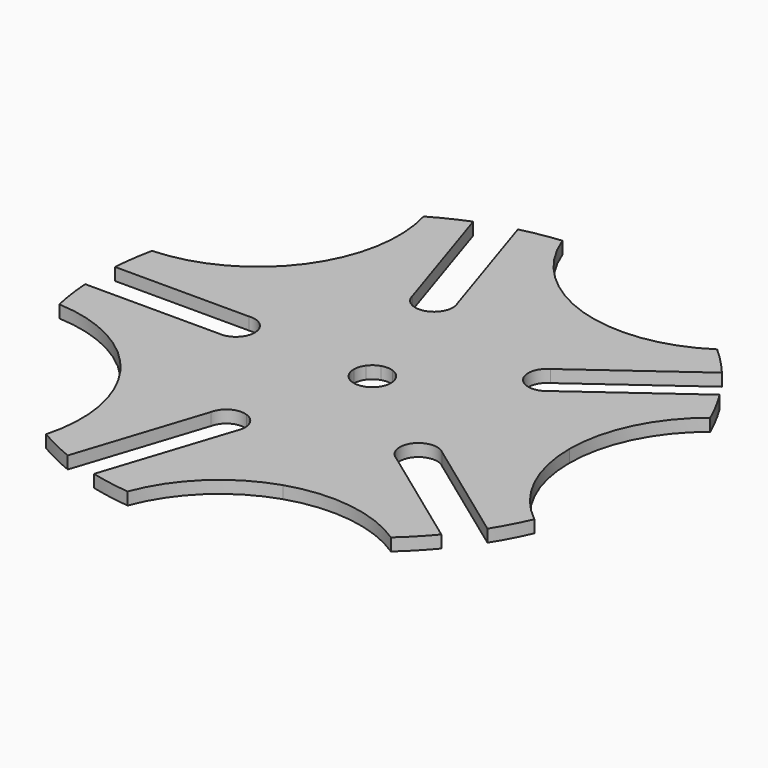
from build123d import *

# Parameters (mm, degrees)
F1_DEPTH = 3.175


# Not quite as in the source:
# - a length typed as a fraction of an inch, garbled in the dataset ("3 / 203.2 mm" for 3/8 in), is restored


with BuildPart() as f1:
    # F0 (on Top) → F1 (new body)
    with BuildSketch(Plane.XY):
        with BuildLine():
            ThreePointArc((-4.7624995714, 0.0020204955), (-4.528844398, 1.4734227733), (-3.8519931198, 2.800634795))
            Line((-3.8519931198, 2.800634795), (-40.7900391434, 29.6568553891))
            ThreePointArc((-40.7900391434, 29.6568553891), (-52.8581727457, 19.1196962374), (-68.3027796686, 14.8610945149))
            ThreePointArc((-68.3027796686, 14.8610945149), (-69.202037382, 9.8589990779), (-69.7354707037, 4.8047857774))
            Line((-69.7354707037, 4.8047857774), (-35.4708737874, 4.7902489857))
            ThreePointArc((-35.4708737874, 4.7902489857), (-31.7421994573, 3.5901618172), (-30.1466961845, 0.012789768))
            Line((-30.1466961845, 0.012789768), (-4.7624995714, 0.0020204955))
        make_face()
        with BuildLine():
            ThreePointArc((-3.8519931198, 2.800634795), (-2.7981829099, 3.853774598), (-1.4705404248, 4.5297811326))
            Line((-1.4705404248, 4.5297811326), (-9.3085437064, 28.6735848558))
            ThreePointArc((-9.3085437064, 28.6735848558), (-13.2035838045, 29.0881739368), (-15.4950023114, 32.2650627762))
            Line((-15.4950023114, 32.2650627762), (-26.0750504874, 64.8553280982))
            ThreePointArc((-26.0750504874, 64.8553280982), (-30.7184565015, 62.789316534), (-35.1994748016, 60.3913802983))
            ThreePointArc((-35.1994748016, 60.3913802983), (-34.4878638746, 44.3862192082), (-40.7900391434, 29.6568553891))
            Line((-40.7900391434, 29.6568553891), (-3.8519931198, 2.800634795))
        make_face()
        with BuildLine():
            ThreePointArc((-1.4705404248, 4.5297811326), (0.0010102478, 4.7624998929), (1.4724620567, 4.5291568466))
            Line((1.4724620567, 4.5291568466), (15.5923915392, 47.9607515681))
            ThreePointArc((15.5923915392, 47.9607515681), (1.8403043285, 56.1797338033), (-6.9847818286, 69.5509501261))
            ThreePointArc((-6.9847818286, 69.5509501261), (-12.0198259563, 68.8596080777), (-16.9913293895, 67.8042518299))
            Line((-16.9913293895, 67.8042518299), (-6.4112812135, 35.213986508))
            ThreePointArc((-6.4112812135, 35.213986508), (-6.3997434798, 31.296961061), (-9.3085437064, 28.6735848558))
            Line((-9.3085437064, 28.6735848558), (-1.4705404248, 4.5297811326))
        make_face()
        with BuildLine():
            ThreePointArc((1.4724620567, 4.5291568466), (2.7998176259, 3.8525871193), (3.8531809453, 2.7990003309))
            Line((3.8531809453, 2.7990003309), (24.390695172, 17.7177155255))
            ThreePointArc((24.390695172, 17.7177155255), (23.5807088667, 21.5500964639), (25.893485986, 24.7114701318))
            Line((25.893485986, 24.7114701318), (53.6158384941, 44.8493445127))
            ThreePointArc((53.6158384941, 44.8493445127), (50.2154123333, 48.626476377), (46.5495312326, 52.1465529318))
            ThreePointArc((46.5495312326, 52.1465529318), (31.5485727352, 46.5213581982), (15.5923915392, 47.9607515681))
            Line((15.5923915392, 47.9607515681), (1.4724620567, 4.5291568466))
        make_face()
        with BuildLine():
            Line((24.390695172, 17.7177155255), (3.8531809453, 2.7990003309))
            ThreePointArc((3.8531809453, 2.7990003309), (4.5294690915, 1.4715012738), (4.7625, 0))
            Line((4.7625, 0), (50.4317, 0))
            ThreePointArc((50.4317, 0), (53.9961373847, 15.6194224529), (63.9836925433, 28.1462063014))
            ThreePointArc((63.9836925433, 28.1462063014), (61.7694966371, 32.7208057029), (59.2287671577, 37.1224323236))
            Line((59.2287671577, 37.1224323236), (31.5064146496, 16.9845579428))
            ThreePointArc((31.5064146496, 16.9845579428), (27.7848747553, 15.7625259109), (24.390695172, 17.7177155255))
        make_face()
        with BuildLine():
            Line((50.4317, 0), (4.7625, 0))
            ThreePointArc((4.7625, 0), (3.8519931198, -2.800634795), (1.4686185281, -4.5304046032))
            Line((1.4686185281, -4.5304046032), (15.5516911338, -47.9739644784))
            ThreePointArc((15.5516911338, -47.9739644784), (31.509087914, -46.5481104778), (46.5052680226, -52.1860315294))
            ThreePointArc((46.5052680226, -52.1860315294), (50.1741345955, -48.6690667492), (53.5777644361, -44.8948215128))
            Line((53.5777644361, -44.8948215128), (25.8725089337, -24.7334319103))
            ThreePointArc((25.8725089337, -24.7334319103), (24.3756528753, -17.7384047006), (31.491991877, -17.0112850838))
            Line((31.491991877, -17.0112850838), (59.1972473794, -37.1726746864))
            ThreePointArc((59.1972473794, -37.1726746864), (61.7556092427, -32.7470085305), (63.9836925433, -28.1462063014))
            ThreePointArc((63.9836925433, -28.1462063014), (53.9961373847, -15.6194224529), (50.4317, 0))
        make_face()
        with BuildLine():
            ThreePointArc((1.4686185281, -4.5304046032), (-0.0030307432, -4.7624990357), (-1.4743834236, -4.5285317455))
            Line((-1.4743834236, -4.5285317455), (-9.3328699489, -28.6656762162))
            ThreePointArc((-9.3328699489, -28.6656762162), (-6.4262967093, -31.2915195998), (-6.4411580428, -35.208533847))
            Line((-6.4411580428, -35.208533847), (-17.0488553147, -67.7898102453))
            ThreePointArc((-17.0488553147, -67.7898102453), (-12.078249143, -68.8493844437), (-7.0437934329, -69.5449984881))
            ThreePointArc((-7.0437934329, -69.5449984881), (1.7926350508, -56.1812750817), (15.5516911338, -47.9739644784))
            Line((15.5516911338, -47.9739644784), (1.4686185281, -4.5304046032))
        make_face()
        with BuildLine():
            ThreePointArc((-1.4743834236, -4.5285317455), (-2.801451838, -3.851398947), (-3.8543680773, -2.797365363))
            Line((-3.8543680773, -2.797365363), (-40.8151883603, -29.6222342844))
            ThreePointArc((-40.8151883603, -29.6222342844), (-34.5255132545, -44.3569402094), (-35.2507043361, -60.3614917348))
            ThreePointArc((-35.2507043361, -60.3614917348), (-30.7717223028, -62.7632292601), (-26.130070975, -64.8331800198))
            Line((-26.130070975, -64.8331800198), (-15.5223737031, -32.2519036214))
            ThreePointArc((-15.5223737031, -32.2519036214), (-13.2282604246, -29.0769601987), (-9.3328699489, -28.6656762162))
            Line((-9.3328699489, -28.6656762162), (-1.4743834236, -4.5285317455))
        make_face()
        with BuildLine():
            ThreePointArc((-3.8543680773, -2.797365363), (-4.5300929698, -1.4695795095), (-4.7624995714, 0.0020204955))
            Line((-4.7624995714, 0.0020204955), (-30.1466961845, 0.012789768))
            ThreePointArc((-30.1466961845, 0.012789768), (-31.7452342902, -3.5632272058), (-35.4749255544, -4.7601501548))
            Line((-35.4749255544, -4.7601501548), (-69.7395224707, -4.7456133631))
            ThreePointArc((-69.7395224707, -4.7456133631), (-69.210377851, -9.8002774634), (-68.3153647492, -14.8031341217))
            ThreePointArc((-68.3153647492, -14.8031341217), (-52.874376818, -19.0748390906), (-40.8151883603, -29.6222342844))
            Line((-40.8151883603, -29.6222342844), (-3.8543680773, -2.797365363))
        make_face()
    extrude(amount=F1_DEPTH)


solid = f1.part
